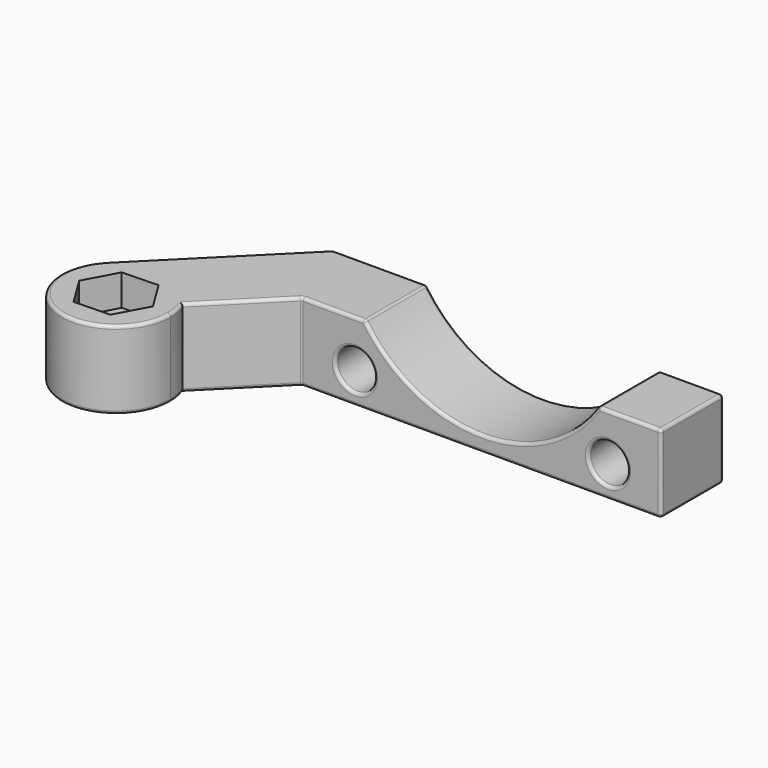
from build123d import *

# Parameters (mm, degrees)
F0_R     = 1.5
F1_DEPTH = 5
F2_R     = 9
F2_R_2   = 1.25
F3_DEPTH = 15
F4_R     = 0.2
F5_START = 3
F5_DEPTH = 2


# Not quite as in the source:
# - a feature names something its author has since deleted; it is built from what else it names


with BuildPart() as f1:
    # F0 (on Top) → F1 (new body)
    with BuildSketch(Plane.XY):
        with BuildLine():
            Line((22.8421047838, 2.0430730569), (22.8421047838, 7.0430730569))
            Line((22.8421047838, 7.0430730569), (-2.1578952162, 7.0430730569))
            Line((-2.1578952162, 7.0430730569), (-10.1578952162, -0.9569269431))
            ThreePointArc((-10.1578952162, -0.9569269431), (-6.9413010441, -0.0112962127), (-4.4053153311, -2.2043470579))
            Line((-4.4053153311, -2.2043470579), (-0.1578952162, 2.0430730569))
            Line((-0.1578952162, 2.0430730569), (22.8421047838, 2.0430730569))
        make_face()
        with BuildLine():
            ThreePointArc((-4.4053153311, -2.2043470579), (-6.9413010441, -0.0112962127), (-10.1578952162, -0.9569269431))
            ThreePointArc((-10.1578952162, -0.9569269431), (-9.0224134954, -6.665379041), (-4.1830214821, -3.4318006772))
            ThreePointArc((-4.1830214821, -3.4318006772), (-4.2390432934, -2.8080906198), (-4.4053153311, -2.2043470579))
        make_face()
        Polygon((-6.5854344834, -1.3998961239), (-5.3745470215, -3.3663866243), (-6.4721340202, -5.3982911776), (-8.7806084808, -5.4637052305), (-9.9914959426, -3.4972147302), (-8.893908944, -1.4653101769), align=None, mode=Mode.SUBTRACT)
        Polygon((-6.4721340202, -5.3982911776), (-5.3745470215, -3.3663866243), (-6.5854344834, -1.3998961239), (-8.893908944, -1.4653101769), (-9.9914959426, -3.4972147302), (-8.7806084808, -5.4637052305), align=None)
        with Locations((-7.6830214821, -3.4318006772)):
            Circle(F0_R, mode=Mode.SUBTRACT)
    extrude(amount=F1_DEPTH)

    # F2 (on Front) → F3 (cut)
    with BuildSketch(Plane.XZ):
        with Locations((11.3421047838, 10)):
            Circle(F2_R)
        with Locations((19.4421047838, 2)):
            Circle(F2_R_2)
        with Locations((3.2421047838, 2)):
            Circle(F2_R_2)
    extrude(amount=-F3_DEPTH, mode=Mode.SUBTRACT)

    # F4
    f4_edges = [f1.edges().sort_by_distance(p)[0] for p in [
        (20.833762, 7.043073, 5),
        (11.342105, 7.043073, 1),
        (11.342105, 2.043073, 0),
        (22.842105, 2.043073, 2.5),
        (20.833762, 2.043073, 5),
        (11.342105, 2.043073, 1),
        (1.850447, 2.043073, 5),
        (-0.157895, 2.043073, 2.5),
        (1.992105, 2.043073, 2),
        (18.192105, 2.043073, 2),
        (-6.183021, -3.431801, 2.5),
        (-9.183021, -3.431801, 0),
        (-9.183021, -3.431801, 5),
        (22.842105, 4.543073, 5),
        (-2.281605, -0.080637, 5),
        (-8.424742, -6.852305, 5),
        (-6.157895, 3.043073, 5),
        (0.850447, 7.043073, 5),
        (3.85879, 4.543073, 5),
        (22.842105, 4.543073, 0),
        (10.342105, 7.043073, 0),
        (-6.157895, 3.043073, 0),
        (-8.424742, -6.852305, 0),
        (-2.281605, -0.080637, 0),
        (18.82542, 4.543073, 5),
        (20.692105, 4.543073, 2),
        (18.192105, 7.043073, 2),
        (22.842105, 7.043073, 2.5),
        (-2.157895, 7.043073, 2.5),
        (1.992105, 7.043073, 2),
        (4.492105, 4.543073, 2),
    ]]
    fillet(f4_edges, radius=F4_R)

    # F0 (on Top) → F5 (cut)
    with BuildSketch(Plane.XY.offset(F5_START)):
        Polygon((-6.4721340202, -5.3982911776), (-5.3745470215, -3.3663866243), (-6.5854344834, -1.3998961239), (-8.893908944, -1.4653101769), (-9.9914959426, -3.4972147302), (-8.7806084808, -5.4637052305), align=None)
        with Locations((-7.6830214821, -3.4318006772)):
            Circle(F0_R, mode=Mode.SUBTRACT)
    extrude(amount=F5_DEPTH, mode=Mode.SUBTRACT)


solid = f1.part
